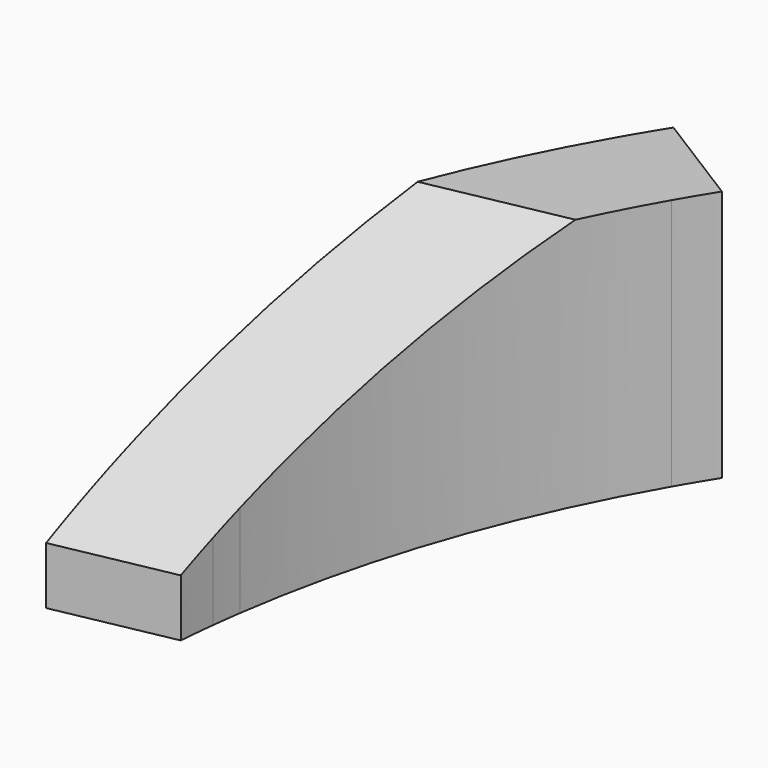
from build123d import *

# Parameters (mm, degrees)
F0_R        = 1.5
F1_DEPTH    = 22
F2_T1_DEPTH = 165.5952281179
F3_DEPTH    = 10


# Not quite as in the source:
# - a fillet or chamfer that OpenCascade refuses, or shapes differently, is made with other operations: its cross-section is extruded or revolved along the edge and cut away or added


with BuildPart() as f1:
    # F0 (on Top) → F1 (new body)
    with BuildSketch(Plane.XY):
        with BuildLine():
            ThreePointArc((-92.2088082298, 7.3338724312), (-92.0714667591, 8.8935374755), (-91.9077462525, 10.4506544671))
            Line((-91.9077462525, 10.4506544671), (-102.1523712509, 8.4346338282))
            ThreePointArc((-102.1523712509, 8.4346338282), (-102.2684274731, 6.8861267905), (-102.3610115463, 5.3360392827))
            Line((-102.3610115463, 5.3360392827), (-92.2088082298, 7.3338724312))
        make_face()
        with BuildLine():
            ThreePointArc((-91.5835416646, 12.9886448933), (-87.4986604127, 30.0039068455), (-80.2824351959, 45.9454089003))
            Line((-80.2824351959, 45.9454089003), (-88.9616173792, 50.9124801328))
            ThreePointArc((-88.9616173792, 50.9124801328), (-96.9579750519, 33.2475724504), (-101.4844650878, 14.3928227196))
            Line((-101.4844650878, 14.3928227196), (-91.5835416646, 12.9886448933))
        make_face()
        with Locations((-94.0054339813, 25.8694488148)):
            Circle(F0_R, mode=Mode.SUBTRACT)
        with Locations((-85.5445299814, 46.7801602206)):
            Circle(F0_R, mode=Mode.SUBTRACT)
        with BuildLine():
            ThreePointArc((-80.2824351959, 45.9454089003), (-79.3561481615, 47.5273789407), (-78.3986924261, 49.0906816603))
            Line((-78.3986924261, 49.0906816603), (-86.8742267425, 54.3977823804))
            ThreePointArc((-86.8742267425, 54.3977823804), (-87.935191206, 52.6654739613), (-88.9616173792, 50.9124801328))
            Line((-88.9616173792, 50.9124801328), (-80.2824351959, 45.9454089003))
        make_face()
        with BuildLine():
            ThreePointArc((-91.9077462525, 10.4506544671), (-91.7544196986, 11.720770699), (-91.5835416646, 12.9886448933))
            Line((-91.5835416646, 12.9886448933), (-101.4844650878, 14.3928227196))
            ThreePointArc((-101.4844650878, 14.3928227196), (-101.8619913522, 11.4186127778), (-102.1523712509, 8.4346338282))
            Line((-102.1523712509, 8.4346338282), (-91.9077462525, 10.4506544671))
        make_face()
        with Locations((-85.5445299814, 46.7801602206)):
            Circle(F0_R)
        with Locations((-94.0054339813, 25.8694488148)):
            Circle(F0_R)
    extrude(amount=F1_DEPTH)

    # F2: chamfer of 17 x 30 on 1 edges, made by hand

    # F2_s2 → F2_t1 (cut)
    with BuildSketch(Plane(origin=(-173.6973169445, -34.1815709152, 0), x_dir=(0, 0, 1), z_dir=(0.9811820369, 0.1930849823, 0))):
        Polygon((5, -25), (22, -55), (22, -25), align=None)
    extrude(amount=F2_T1_DEPTH, mode=Mode.SUBTRACT)

    # F0 (on Top) → F3 (cut)
    with BuildSketch(Plane.XY):
        with Locations((-85.5445299814, 46.7801602206)):
            Circle(F0_R)
        with Locations((-94.0054339813, 25.8694488148)):
            Circle(F0_R)
    extrude(amount=F3_DEPTH, mode=Mode.SUBTRACT)


solid = f1.part
